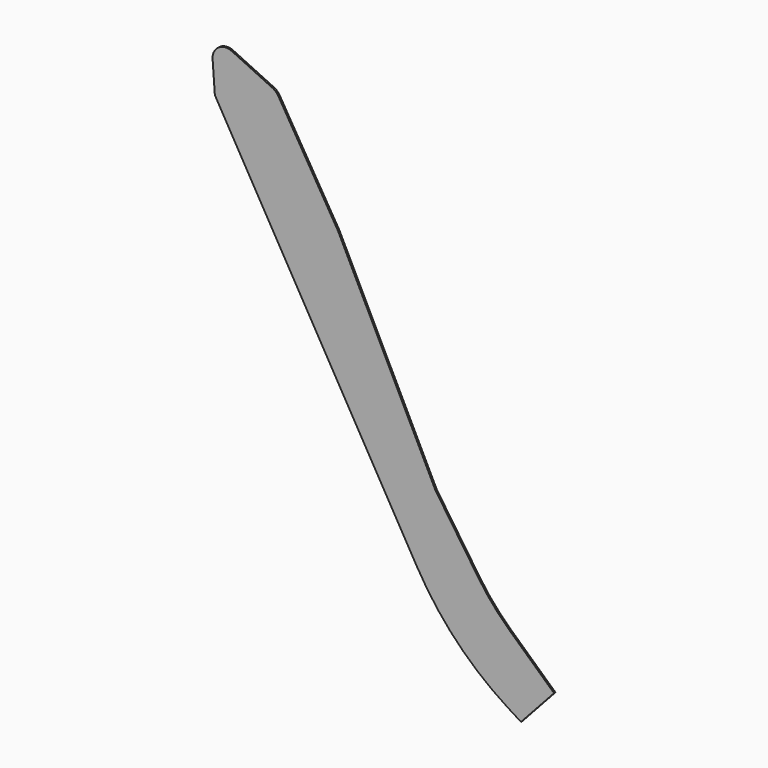
from build123d import *

# Parameters (mm, degrees)
F1_DEPTH = 3.175


# Not quite as in the source:
# - ends of sketch curves that miss each other by under 0.0002 mm in the source are joined


with BuildPart() as f1:
    # F0 (on Front) → F1 (new body)
    with BuildSketch(Plane.XZ):
        with BuildLine():
            Line((256.8526232, -464.2309994), (318.5212324, -396.9739076))
            Line((318.5212324, -396.9739076), (235.5036438, -320.8543748))
            ThreePointArc((235.5036438, -320.8543748), (204.8703266123, -289.3256959733), (178.0726202767, -254.4783059859))
            Line((178.0726202767, -254.4783059859), (97.204276, -135.7211662))
            Line((97.204276, -135.7211662), (-84.3345278, 230.8220174))
            Line((-84.3345278, 230.8220174), (-195.8067712, 416.2626422))
            ThreePointArc((-195.8067712, 416.2626422), (-200.5384813212, 422.0145789545), (-206.7351977857, 426.1467211829))
            Line((-206.7351977857, 426.1467211829), (-282.2801314, 461.8011846))
            ThreePointArc((-282.2801314, 461.8011846), (-307.4924345817, 459.774434742), (-318.4536458896, 436.9792648454))
            Line((-318.4536458896, 436.9792648454), (-314.4572832, 382.307084))
            ThreePointArc((-314.4572832, 382.307084), (-313.9285810002, 379.4952234768), (-312.7838670978, 376.873066496))
            Line((-312.7838670978, 376.873066496), (63.4258828, -273.3887852))
            ThreePointArc((63.4258828, -273.3887852), (137.2742586369, -371.4240291313), (232.4799240247, -448.8861008552))
            Line((232.4799240247, -448.8861008552), (256.8526232, -464.2309994))
        make_face()
    extrude(amount=F1_DEPTH)


solid = f1.part
